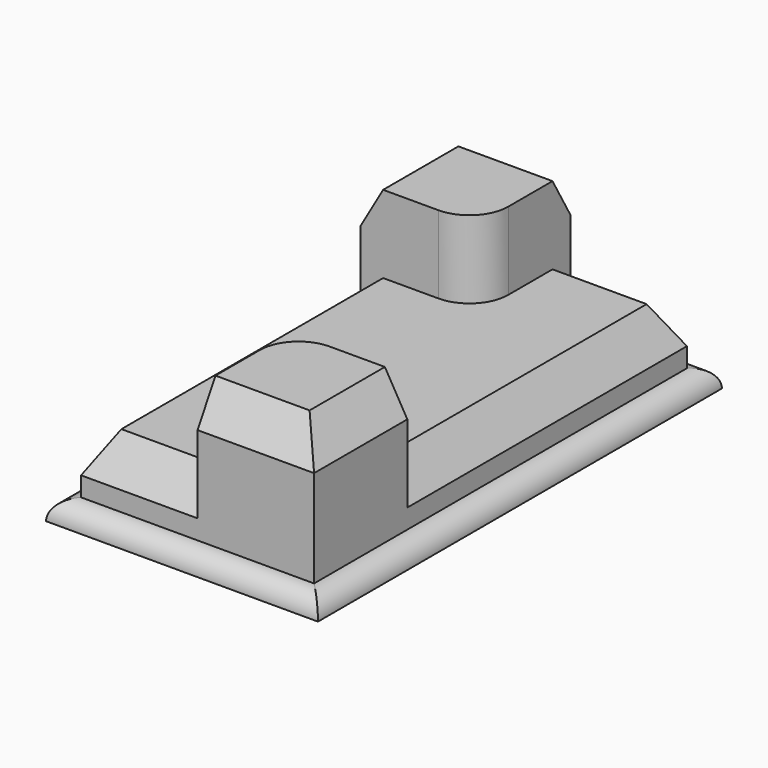
from build123d import *

# Parameters (mm, degrees)
F0_W       = 88.9
F0_H       = 165.1
F1_DEPTH   = 6.35
F2_DEPTH   = 25.4
F3_DEPTH   = 50.8
F4_R       = 6.34999
F5_SIZE2   = 12.7
F5_SIZE    = 7.3323484187
F6_SIZE2   = 12.7
F6_SIZE    = 7.3323484187
F6_2_SIZE2 = 12.7
F6_2_SIZE  = 7.3323484187


# Not quite as in the source:
# - a fillet or chamfer is up to 0.001 mm smaller than in the source, because OpenCascade refuses the exact size


with BuildPart() as f1:
    # F0 (on Top) → F1 (new body)
    with BuildSketch(Plane.XY):
        with Locations((-15.4908802681, 0.7453764391)):
            Rectangle(F0_W, F0_H)
        Polygon((-53.5908802681, 38.8453764391), (-53.5908802681, 76.9453764391), (-15.4908802681, 76.9453764391), (22.6091197319, 76.9453764391), (22.6091197319, -37.3546235609), (22.6091197319, -75.4546235609), (-15.4908802681, -75.4546235609), (-53.5908802681, -75.4546235609), align=None, mode=Mode.SUBTRACT)
    extrude(amount=F1_DEPTH)

    # F0 (on Top) → F2 (join)
    with BuildSketch(Plane.XY):
        with BuildLine():
            Line((22.6091197319, 76.9453764391), (-15.4908802681, 76.9453764391))
            Line((-15.4908802681, 76.9453764391), (-15.4908802681, 51.5453764391))
            ThreePointArc((-15.4908802681, 51.5453764391), (-19.2106241471, 42.5651203181), (-28.1908802681, 38.8453764391))
            Line((-28.1908802681, 38.8453764391), (-53.5908802681, 38.8453764391))
            Line((-53.5908802681, 38.8453764391), (-53.5908802681, -75.4546235609))
            Line((-53.5908802681, -75.4546235609), (-15.4908802681, -75.4546235609))
            Line((-15.4908802681, -75.4546235609), (-15.4908802681, -50.0546235609))
            ThreePointArc((-15.4908802681, -50.0546235609), (-11.7711363892, -41.0743674398), (-2.7908802681, -37.3546235609))
            Line((-2.7908802681, -37.3546235609), (22.6091197319, -37.3546235609))
            Line((22.6091197319, -37.3546235609), (22.6091197319, 76.9453764391))
        make_face()
    extrude(amount=F2_DEPTH)

    # F0 (on Top) → F3 (join)
    with BuildSketch(Plane.XY):
        with BuildLine():
            Line((-15.4908802681, 76.9453764391), (-53.5908802681, 76.9453764391))
            Line((-53.5908802681, 76.9453764391), (-53.5908802681, 38.8453764391))
            Line((-53.5908802681, 38.8453764391), (-28.1908802681, 38.8453764391))
            ThreePointArc((-28.1908802681, 38.8453764391), (-19.2106241471, 42.5651203181), (-15.4908802681, 51.5453764391))
            Line((-15.4908802681, 51.5453764391), (-15.4908802681, 76.9453764391))
        make_face()
        with BuildLine():
            Line((22.6091197319, -75.4546235609), (22.6091197319, -37.3546235609))
            Line((22.6091197319, -37.3546235609), (-2.7908802681, -37.3546235609))
            ThreePointArc((-2.7908802681, -37.3546235609), (-11.7711363892, -41.0743674398), (-15.4908802681, -50.0546235609))
            Line((-15.4908802681, -50.0546235609), (-15.4908802681, -75.4546235609))
            Line((-15.4908802681, -75.4546235609), (22.6091197319, -75.4546235609))
        make_face()
    extrude(amount=F3_DEPTH)

    # F4 (radius 6.35 in the source; OpenCascade refuses exactly that, so slightly less here)
    f4_edges = [f1.edges().sort_by_distance(p)[0] for p in [
        (28.95912, 0.745376, 6.35),
        (-15.49088, -81.804624, 6.35),
        (-59.94088, 0.745376, 6.35),
        (-15.49088, 83.295376, 6.35),
    ]]
    fillet(f4_edges, radius=F4_R)

    # F5
    f5_edges = [f1.edges().sort_by_distance(p)[0] for p in [
        (-34.54088, -75.454624, 25.4),
        (-53.59088, -18.304624, 25.4),
        (22.60912, 19.795376, 25.4),
        (3.55912, 76.945376, 25.4),
    ]]
    f5_side = f1.faces().sort_by_distance((-15.49088, 0.745376, 25.4))[0]
    chamfer(f5_edges, length=F5_SIZE, length2=F5_SIZE2, reference=f5_side)

    # F6
    f6_edges = [f1.edges().sort_by_distance(p)[0] for p in [
        (-34.54088, 76.945376, 50.8),
        (-53.59088, 57.895376, 50.8),
    ]]
    f6_side = f1.faces().sort_by_distance((-34.936922, 58.291419, 50.8))[0]
    chamfer(f6_edges, length=F6_SIZE, length2=F6_SIZE2, reference=f6_side)

    # F6#2
    f6_2_edges = [f1.edges().sort_by_distance(p)[0] for p in [
        (22.60912, -56.404624, 50.8),
        (3.55912, -75.454624, 50.8),
    ]]
    f6_2_side = f1.faces().sort_by_distance((3.955162, -56.800666, 50.8))[0]
    chamfer(f6_2_edges, length=F6_2_SIZE, length2=F6_2_SIZE2, reference=f6_2_side)


solid = f1.part
